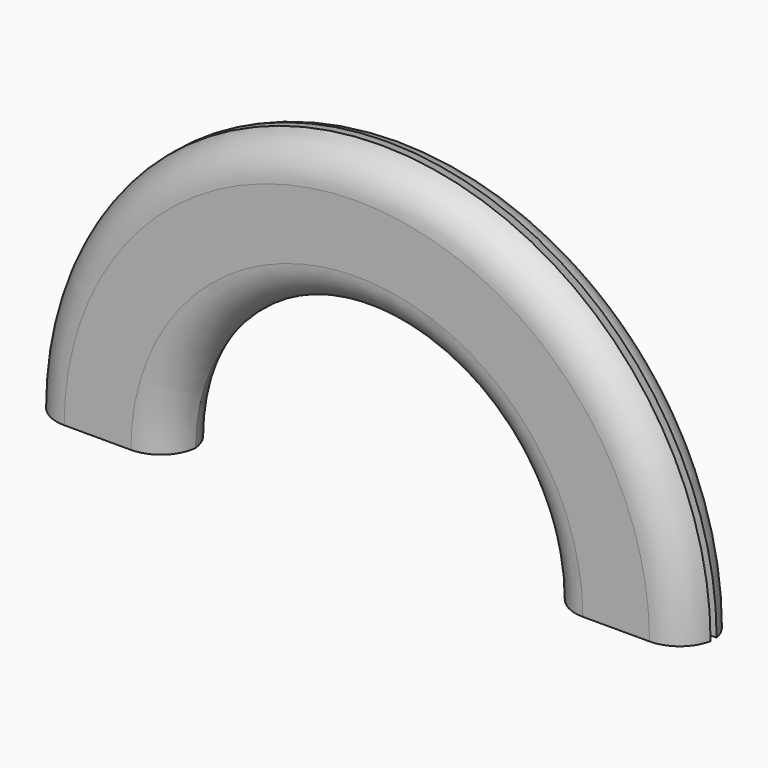
from build123d import *

# Parameters (mm, degrees)
F3_T2_ANGLE = 212.1305431318
F3_T4_ANGLE = 212.1305431318
F3_T6_ANGLE = 237.3879219603
F3_T8_ANGLE = 237.3879219603


# Not quite as in the source:
# - a fillet or chamfer that OpenCascade refuses, or shapes differently, is made with other operations: its cross-section is extruded or revolved along the edge and cut away or added


with BuildPart() as f2:
    # F2: sweep along a path in F0
    with BuildLine(Plane.XZ) as f2_path:
        ThreePointArc((-12.7, 0), (0, 12.7), (12.7, 0))
    # F1 (on Top) → F2 (sweep)
    with BuildSketch(Plane.XY):
        with BuildLine():
            Line((-12.7, -4.572), (-12.7, 0))
            Line((-12.7, 0), (-22.225, 0))
            Line((-22.225, 0), (-22.225, -2.032))
            Line((-22.225, -2.032), (-20.701, -2.032))
            Line((-20.701, -2.032), (-20.701, -1.651))
            Line((-20.701, -1.651), (-14.732, -1.651))
            Line((-14.732, -1.651), (-14.732, -2.921))
            Line((-14.732, -2.921), (-20.5930953096, -2.921))
            ThreePointArc((-20.5930953096, -2.921), (-20.6693954479, -2.8893954479), (-20.701, -2.8130953096))
            Line((-20.701, -2.8130953096), (-20.701, -2.54))
            Line((-20.701, -2.54), (-22.225, -2.54))
            Line((-22.225, -2.54), (-22.225, -4.572))
            Line((-22.225, -4.572), (-12.7, -4.572))
        make_face()
    sweep(path=f2_path.line)

    # F3: fillet of radius 2.54 on 4 edges, made by hand

    # F3_s1 → F3_t2 (revolve, cut)
    with BuildSketch(Plane(origin=(0, 0, 0), x_dir=(0, 1, 0), z_dir=(0.2767322496, 0, -0.9609470651))):
        with BuildLine():
            ThreePointArc((-2.54, -22.225), (-3.9994755399, -21.3427554727), (-4.572, -19.7363184213))
            Line((-4.572, -19.7363184213), (-4.572, -22.225))
            Line((-4.572, -22.225), (-2.54, -22.225))
        make_face()
    revolve(axis=Axis((0, -4.572, 0), (0, 1, 0)), revolution_arc=F3_T2_ANGLE, mode=Mode.SUBTRACT)

    # F3_s3 → F3_t4 (revolve, cut)
    with BuildSketch(Plane(origin=(0, 0, 0), x_dir=(0, 1, 0), z_dir=(0.2767322496, 0, -0.9609470651))):
        with BuildLine():
            ThreePointArc((0, -19.7363184213), (-0.5725244601, -21.3427554727), (-2.032, -22.225))
            Line((-2.032, -22.225), (0, -22.225))
            Line((0, -22.225), (0, -19.7363184213))
        make_face()
    revolve(axis=Axis((0, 0, 0), (0, 1, 0)), revolution_arc=F3_T4_ANGLE, mode=Mode.SUBTRACT)

    # F3_s5 → F3_t6 (revolve, cut)
    with BuildSketch(Plane(origin=(0, 0, 0), x_dir=(0, 1, 0), z_dir=(0.4801310429, 0, -0.8771967748))):
        with BuildLine():
            ThreePointArc((-2.032, -12.7), (-3.8280512242, -13.4439487758), (-4.572, -15.24))
            Line((-4.572, -15.24), (-4.572, -12.7))
            Line((-4.572, -12.7), (-2.032, -12.7))
        make_face()
    revolve(axis=Axis((0, -4.572, 0), (0, 1, 0)), revolution_arc=F3_T6_ANGLE, mode=Mode.SUBTRACT)

    # F3_s7 → F3_t8 (revolve, cut)
    with BuildSketch(Plane(origin=(0, 0, 0), x_dir=(0, 1, 0), z_dir=(0.4801310429, 0, -0.8771967748))):
        with BuildLine():
            ThreePointArc((-2.54, -12.7), (-0.7439487758, -13.4439487758), (0, -15.24))
            Line((0, -15.24), (0, -12.7))
            Line((0, -12.7), (-2.54, -12.7))
        make_face()
    revolve(axis=Axis((0, 0, 0), (0, 1, 0)), revolution_arc=F3_T8_ANGLE, mode=Mode.SUBTRACT)


solid = f2.part
